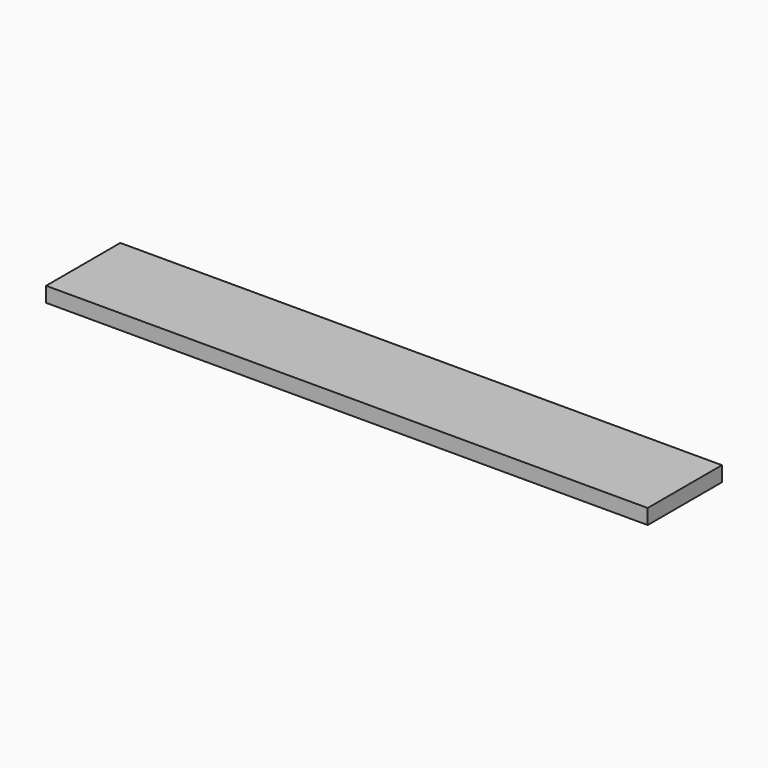
from build123d import *

# Parameters (mm, degrees)
F1_W     = 234.95
F1_H     = 38.1
F2_DEPTH = 762


# Not quite as in the source:
# - a variable given as a bare number and used for a length is read in inches; the dataset says mm whatever the document's units were


with BuildPart() as f2:
    # F1 (on Right) → F2 (new body, symmetric)
    with BuildSketch(Plane.YZ):
        with Locations((6.7235322315, 0)):
            Rectangle(F1_W, F1_H)
    extrude(amount=F2_DEPTH, both=True)


solid = f2.part
